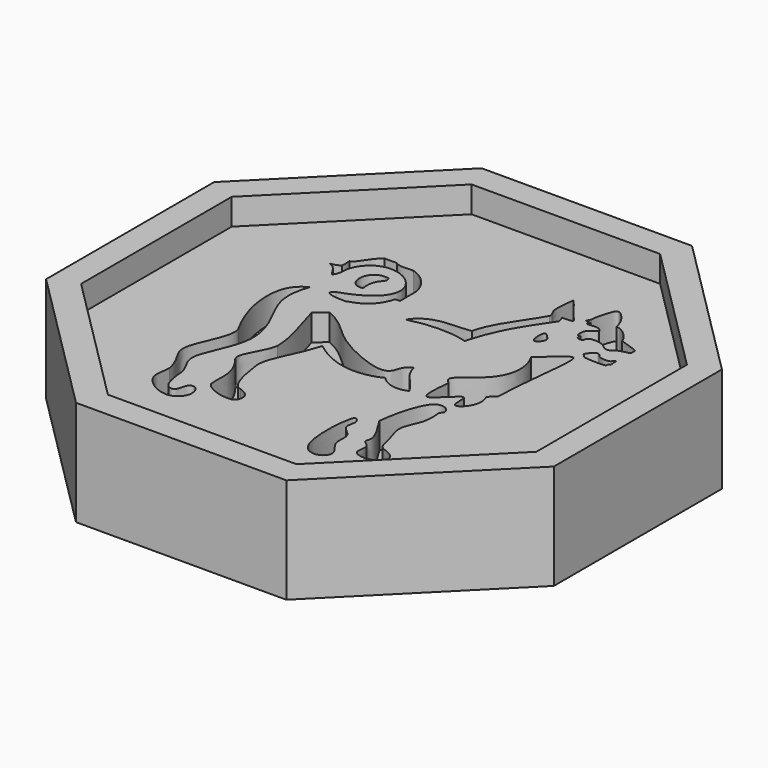
from build123d import *

# Parameters (mm, degrees)
F1_DEPTH = 25.4
F3_DEPTH = 6.35
F5_DEPTH = 6.35


with BuildPart() as f1:
    # F0 (on Top) → F1 (new body)
    with BuildSketch(Plane.XY):
        Polygon((-61.3372846899, 25.3607087968), (-61.3047391097, -25.4392807779), (-25.3607087968, -61.3372846899), (25.4392807779, -61.3047391097), (61.3372846899, -25.3607087968), (61.3047391097, 25.4392807779), (25.3607087968, 61.3372846899), (-25.4392807779, 61.3047391097), align=None)
    extrude(amount=F1_DEPTH)

    # F2 (on face) → F3 (cut)
    with BuildSketch(Plane.XY.offset(25.4)):
        Polygon((-54.9856008905, 22.734521413), (-54.9564255154, -22.8049569991), (-22.734521413, -54.9856008905), (22.8049569991, -54.9564255154), (54.9856008905, -22.734521413), (54.9564255154, 22.8049569991), (22.734521413, 54.9856008905), (-22.8049569991, 54.9564255154), align=None)
    extrude(amount=-F3_DEPTH, mode=Mode.SUBTRACT)

    # F4 (on face) → F5 (cut)
    with BuildSketch(Plane.XY.offset(19.05)):
        with BuildLine():
            add(Edge.make_bspline(
                [(-28.0372798443, 19.2676149309), (-28.8987054179, 20.3235540539), (-29.2879249901, 21.9352524728), (-31.1219263822, 22.5187968463)],
                knots=[0, 0, 0, 0, 4.4816546175, 4.4816546175, 4.4816546175, 4.4816546175], degree=3))
            add(Edge.make_bspline(
                [(-28.0372798443, 19.2676149309), (-26.9745588303, 20.3046072274), (-27.197111398, 22.6414259523), (-27.0301960409, 23.2191737741)],
                knots=[0, 0, 0, 0, 4.0778713907, 4.0778713907, 4.0778713907, 4.0778713907], degree=3))
            add(Edge.make_bspline(
                [(-27.0301960409, 23.2191737741), (-22.4121976644, 35.549569875), (-2.2154052276, 20.9722686559), (-22.9129437357, 14.1843669116)],
                knots=[0, 0, 0, 0, 9.9287210449, 9.9287210449, 9.9287210449, 9.9287210449], degree=3))
            add(Edge.make_bspline(
                [(-22.9129437357, 14.1843669116), (-25.3610387444, 12.6264877617), (-21.5219799429, 12.2926570475), (-19.185161218, 12.3482951894)],
                knots=[0, 0, 0, 0, 4.1554207811, 4.1554207811, 4.1554207811, 4.1554207811], degree=3))
            add(Edge.make_bspline(
                [(-19.185161218, 12.3482951894), (-16.6814271361, 13.1272347644), (-13.6213079095, 14.3512832001), (-12.3416194692, 18.8580043614)],
                knots=[0, 0, 0, 0, 9.4451245186, 9.4451245186, 9.4451245186, 9.4451245186], degree=3))
            add(Edge.make_bspline(
                [(-12.3416194692, 18.8580043614), (-11.9706960395, 18.8580043614), (-11.5997726098, 18.8580043614), (-11.22884918, 18.8580043614)],
                knots=[0, 0, 0, 0, 1.1127702892, 1.1127702892, 1.1127702892, 1.1127702892], degree=3))
            add(Edge.make_bspline(
                [(-11.22884918, 18.8580043614), (-11.22884918, 20.5086146792), (-11.22884918, 22.159224997), (-11.22884918, 23.8098353148)],
                knots=[0, 0, 0, 0, 4.9518309534, 4.9518309534, 4.9518309534, 4.9518309534], degree=3))
            add(Edge.make_bspline(
                [(-11.22884918, 23.8098353148), (-11.6183189675, 25.8128233254), (-13.0092836916, 28.7616662681), (-17.0152578503, 30.1526300609)],
                knots=[0, 0, 0, 0, 8.5856607487, 8.5856607487, 8.5856607487, 8.5856607487], degree=3))
            add(Edge.make_bspline(
                [(-17.0152578503, 30.1526300609), (-18.4618607163, 30.1526300609), (-20.2422942966, 29.7075212002), (-21.2994255126, 30.597737059)],
                knots=[0, 0, 0, 0, 4.3072279715, 4.3072279715, 4.3072279715, 4.3072279715], degree=3))
            add(Edge.make_bspline(
                [(-21.2994255126, 30.597737059), (-22.3009195179, 30.597737059), (-23.3024135232, 30.597737059), (-24.3039075285, 30.597737059)],
                knots=[0, 0, 0, 0, 3.004482016, 3.004482016, 3.004482016, 3.004482016], degree=3))
            add(Edge.make_bspline(
                [(-24.3039075285, 30.597737059), (-26.6407262534, 28.9842206985), (-27.4196658283, 25.8684623986), (-28.8662686944, 25.590268895)],
                knots=[0, 0, 0, 0, 6.77420673, 6.77420673, 6.77420673, 6.77420673], degree=3))
            add(Edge.make_bspline(
                [(-28.8662686944, 25.590268895), (-28.8662686944, 24.8484214147), (-28.5880770534, 24.0323897451), (-28.8662686944, 23.364726454)],
                knots=[0, 0, 0, 0, 2.225542441, 2.225542441, 2.225542441, 2.225542441], degree=3))
            add(Edge.make_bspline(
                [(-28.8662686944, 23.364726454), (-29.4782929122, 22.8083413094), (-30.3700404863, 22.6524043828), (-31.1219263822, 22.5187968463)],
                knots=[0, 0, 0, 0, 2.4090638235, 2.4090638235, 2.4090638235, 2.4090638235], degree=3))
        make_face()
        with BuildLine():
            add(Edge.make_bspline(
                [(-28.0008820709, 12.7586783027), (-29.8796463948, 7.5660265069), (-28.0287999384, 2.6821632246), (-26.7683431041, -0.0068068178), (-20.7281608533, -11.1412521717), (-29.5474328001, -23.7696430619), (-26.0852734071, -26.7943696783), (-25.2977338724, -29.1416380778)],
                knots=[0, 0, 0, 0, 0.2225477667, 0.3405641947, 0.5755616363, 0.8292797736, 1, 1, 1, 1], degree=3))
            add(Edge.make_bspline(
                [(-28.0008820709, 12.7586783027), (-29.4725771484, 11.8279191796), (-32.867634998, 9.2120678884), (-32.5076486915, -0.8590882644), (-28.0565619469, -8.8710384443)],
                knots=[0, 0, 0, 0, 0.3407457975, 1, 1, 1, 1], degree=3))
            add(Edge.make_bspline(
                [(-28.0565619469, -8.8710384443), (-26.4949586198, -11.4365298913), (-32.0736885782, -20.3703801564), (-30.4349170995, -24.4972697778), (-28.4926244503, -27.3833730072), (-28.0565638095, -29.6726982143)],
                knots=[0, 0, 0, 0, 0.4345714436, 0.6971037116, 1, 1, 1, 1], degree=3))
            add(Edge.make_bspline(
                [(-28.0565638095, -29.6726982143), (-28.0565638095, -31.237732619), (-29.6389633306, -35.0945037642), (-21.898898007, -39.9078726353), (-18.7092870474, -37.3579747975), (-18.3754581958, -35.6888175011)],
                knots=[0, 0, 0, 0, 0.316261051, 0.6980595292, 1, 1, 1, 1], degree=3))
            add(Edge.make_bspline(
                [(-18.3754581958, -35.6888175011), (-18.2647514631, -34.6924680256), (-18.4831757484, -33.6313286516), (-19.7782164584, -32.3324423498), (-21.4117624362, -33.3148451966), (-21.3484425752, -36.0815248294), (-24.3933898287, -36.1620581292), (-25.0957816794, -32.0893552414), (-25.2977338724, -29.1416380778)],
                knots=[0, 0, 0, 0, 0.1574034873, 0.285836077, 0.4154273106, 0.580633255, 0.7196315018, 1, 1, 1, 1], degree=3))
        make_face()
        with BuildLine():
            add(Edge.make_bspline(
                [(-18.7092870474, 6.9303079508), (-13.8535913481, 4.7580242148), (-11.9416435709, 0.119009405), (7.1841906574, -8.3140862474), (5.5491165258, -1.5267506242), (7.8859366477, -0.8590877987)],
                knots=[0, 0, 0, 0, 0.3593902316, 0.765142193, 1, 1, 1, 1], degree=3))
            add(Edge.make_bspline(
                [(-21.2686602026, 4.7580242148), (-20.4155358175, 5.4821187935), (-19.5624114325, 6.2062133721), (-18.7092870474, 6.9303079508)],
                knots=[0, 0, 0, 0, 3.3569640418, 3.3569640418, 3.3569640418, 3.3569640418], degree=3))
            add(Edge.make_bspline(
                [(-17.8190711886, -9.8725324497), (-17.9303474724, -6.0891113244), (-18.5980126262, -4.3086772785), (-21.2686602026, 4.7580242148)],
                knots=[0, 0, 0, 0, 15.0317281999, 15.0317281999, 15.0317281999, 15.0317281999], degree=3))
            add(Edge.make_bspline(
                [(-20.8235513419, -18.8859757036), (-21.713770926, -16.5491569787), (-18.3754581958, -13.6559531093), (-17.8190711886, -9.8725324497)],
                knots=[0, 0, 0, 0, 9.5010031199, 9.5010031199, 9.5010031199, 9.5010031199], degree=3))
            add(Edge.make_bspline(
                [(-17.9303487142, -29.8653164258), (-18.3754581958, -26.1189863086), (-16.8175771832, -24.0047220141), (-20.8235513419, -18.8859757036)],
                knots=[0, 0, 0, 0, 11.3541421577, 11.3541421577, 11.3541421577, 11.3541421577], degree=3))
            add(Edge.make_bspline(
                [(-17.262686044, -30.6813474745), (-17.4852402674, -30.4093371249), (-17.7077944908, -30.1373267753), (-17.9303487142, -29.8653164258)],
                knots=[0, 0, 0, 0, 1.0543624204, 1.0543624204, 1.0543624204, 1.0543624204], degree=3))
            add(Edge.make_bspline(
                [(-12.2552160174, -28.0106980354), (-11.2932488833, -28.3518757818), (-9.3914477485, -29.2781346218), (-9.8999895977, -32.4848488774), (-12.3449518616, -32.5252296346), (-14.7961370982, -32.1376830066), (-16.3743810316, -31.3027464304), (-17.262686044, -30.6813474745)],
                knots=[0, 0, 0, 0, 0.2134300381, 0.406934161, 0.5873424903, 0.7860112945, 1, 1, 1, 1], degree=3))
            add(Edge.make_bspline(
                [(-15.9273585305, -18.6634231359), (-15.3709752485, -22.780675441), (-14.4807593897, -27.788143605), (-12.2552160174, -28.0106980354)],
                knots=[0, 0, 0, 0, 10.0427176941, 10.0427176941, 10.0427176941, 10.0427176941], degree=3))
            add(Edge.make_bspline(
                [(-11.1424466595, -4.6425093897), (-13.0341565236, -11.096579954), (-16.2611911073, -14.7687252611), (-15.9273585305, -18.6634231359)],
                knots=[0, 0, 0, 0, 14.8149047885, 14.8149047885, 14.8149047885, 14.8149047885], degree=3))
            add(Edge.make_bspline(
                [(6.2167802826, -7.4244360439), (2.5446349755, -9.3161463737), (-4.1319923475, -10.3176408447), (-11.1424466595, -4.6425093897)],
                knots=[0, 0, 0, 0, 17.5807245566, 17.5807245566, 17.5807245566, 17.5807245566], degree=3))
            add(Edge.make_bspline(
                [(6.2167802826, -7.4244360439), (8.4423208609, -9.6499780193), (11.1129721627, -9.7612552345), (13.115959242, -8.7597612292)],
                knots=[0, 0, 0, 0, 7.0272159256, 7.0272159256, 7.0272159256, 7.0272159256], degree=3))
            add(Edge.make_bspline(
                [(7.8859366477, -0.8590877987), (8.7761525065, -4.5312321745), (11.3355256617, -5.5327252485), (13.115959242, -8.7597612292)],
                knots=[0, 0, 0, 0, 9.4749024792, 9.4749024792, 9.4749024792, 9.4749024792], degree=3))
        make_face()
        with BuildLine():
            add(Edge.make_bspline(
                [(-19.9287291616, 18.5597520322), (-20.7218211144, 23.2191737741), (-17.6485870034, 22.9217652231), (-18.6399519444, 24.7062239796)],
                knots=[0, 0, 0, 0, 6.2801324919, 6.2801324919, 6.2801324919, 6.2801324919], degree=3))
            add(Edge.make_bspline(
                [(-18.6399519444, 24.7062239796), (-23.9933300763, 25.8958619088), (-24.3898760527, 17.7666600794), (-19.9287291616, 18.5597520322)],
                knots=[0, 0, 0, 0, 6.2801324919, 6.2801324919, 6.2801324919, 6.2801324919], degree=3))
        make_face()
        with BuildLine():
            add(Edge.make_bspline(
                [(-5.6096651642, 13.6149282611), (-2.6132406574, 18.4601675352), (4.203310702, 17.065346241), (7.0364302956, 17.7666600802)],
                knots=[0, 0, 0, 0, 13.3101693256, 13.3101693256, 13.3101693256, 13.3101693256], degree=3))
            add(Edge.make_bspline(
                [(-5.6096651642, 13.6149282611), (1.4386394164, 15.3351114917), (6.2239428516, 14.3849765882), (8.5040840786, 13.6910192668)],
                knots=[0, 0, 0, 0, 14.1139543548, 14.1139543548, 14.1139543548, 14.1139543548], degree=3))
            add(Edge.make_bspline(
                [(8.5040840786, 13.6910192668), (10.7672957238, 22.0507318154), (14.4973509014, 26.6936998814), (17.3945371062, 31.0881678015)],
                knots=[0, 0, 0, 0, 19.537167967, 19.537167967, 19.537167967, 19.537167967], degree=3))
            add(Edge.make_bspline(
                [(16.957372427, 32.6494723558), (17.1044332286, 31.9786133866), (17.2474763046, 31.7590267708), (17.3945371062, 31.0881678015)],
                knots=[0, 0, 0, 0, 1.6213527895, 1.6213527895, 1.6213527895, 1.6213527895], degree=3))
            add(Edge.make_bspline(
                [(16.957372427, 32.6494723558), (17.6561995983, 32.5662349947), (18.8445488517, 32.710853988), (19.5890592956, 32.8586511932), (19.3132246383, 33.2443414188), (19.1744230688, 33.430121839)],
                knots=[0, 0, 0, 0, 0.4924790738, 0.7397762109, 1, 1, 1, 1], degree=3))
            add(Edge.make_bspline(
                [(14.147025533, 39.4879803061), (16.0163631663, 37.5952757895), (17.3050854355, 35.3228263557), (19.1744230688, 33.430121839)],
                knots=[0, 0, 0, 0, 7.8722535014, 7.8722535014, 7.8722535014, 7.8722535014], degree=3))
            add(Edge.make_bspline(
                [(14.6084949374, 31.7074209452), (14.8813206561, 32.4576937104), (13.1977047154, 33.5858091233), (14.0470692435, 37.3768965245), (14.147025533, 39.4879803061)],
                knots=[0, 0, 0, 0, 0.3731092448, 1, 1, 1, 1], degree=3))
            add(Edge.make_bspline(
                [(7.0364302956, 17.7666600802), (8.159278892, 22.8046998382), (12.0844733902, 27.0605006569), (14.6084949374, 31.7074209452)],
                knots=[0, 0, 0, 0, 15.8644563863, 15.8644563863, 15.8644563863, 15.8644563863], degree=3))
        make_face()
        with BuildLine():
            add(Edge.make_bspline(
                [(22.4148165435, 16.3930356503), (24.2836665154, 18.0725250896), (27.0029173159, 20.549754426), (30.4862581168, 22.5940611271), (27.8906989843, 10.1220104843), (27.6257377118, 0)],
                knots=[0, 0, 0, 0, 0.30682698, 0.451722506, 1, 1, 1, 1], degree=3))
            add(Edge.make_bspline(
                [(16.8506149203, -1.5367978485), (16.2638233056, -1.0676976254), (14.492191998, 0.4182380512), (24.3064990699, 5.4345626379), (24.4445025559, 13.0395053067), (22.4148165435, 16.3930356503)],
                knots=[0, 0, 0, 0, 0.1793899189, 0.5722506166, 1, 1, 1, 1], degree=3))
            add(Edge.make_bspline(
                [(25.9476453066, -1.5367978485), (27.8751199964, -5.0414433062), (21.9399501079, -11.1675266732), (24.2107532041, -0.8994806889), (15.6309805834, -12.4569427437), (16.5765762449, -5.1974706536), (16.8506149203, -1.5367978485)],
                knots=[0, 0, 0, 0, 0.2678703185, 0.4625212705, 0.7285866825, 1, 1, 1, 1], degree=3))
            add(Edge.make_bspline(
                [(27.6257377118, 0), (27.00749288, -0.3945002488), (26.5658901383, -1.1422975998), (25.9476453066, -1.5367978485)],
                knots=[0, 0, 0, 0, 2.2754651717, 2.2754651717, 2.2754651717, 2.2754651717], degree=3))
        make_face()
        with BuildLine():
            add(Edge.make_bspline(
                [(13.1382956089, -25.0052385354), (13.0518203589, -24.3990163752), (12.2797618583, -23.5602785403), (11.1105141174, -24.4906442838), (9.9794661919, -39.7643581614), (16.6902932342, -40.4762091746), (18.5003941614, -37.0816704912), (14.7121952101, -34.3856699364), (16.2425085179, -29.7885953701), (12.1334767397, -28.1036926101), (13.2568177087, -25.8361204735), (13.1382956089, -25.0052385354)],
                knots=[0, 0, 0, 0, 0.070863397, 0.1257912558, 0.3447714787, 0.4684229399, 0.5640410455, 0.6792790888, 0.7964704868, 0.9028753475, 1, 1, 1, 1], degree=3))
        make_face()
        with BuildLine():
            add(Edge.make_bspline(
                [(26.8536079675, -34.3594290316), (27.2714490269, -33.9821628087), (27.5024453322, -32.7005899885), (26.7680687179, -31.4202354743), (24.9856919844, -30.5617172645), (22.9394136433, -29.949434594), (22.5963966728, -25.9982062628), (20.4523282947, -21.7454574747), (23.4664017858, -17.1000129061), (23.2859773282, -13.901970828), (23.1107082218, -12.2754126787)],
                knots=[0, 0, 0, 0, 0.0942279731, 0.180240306, 0.2818144223, 0.3812242085, 0.5202976451, 0.6764919854, 0.8400809199, 1, 1, 1, 1], degree=3))
            add(Edge.make_bspline(
                [(23.1107082218, -12.2754126787), (23.3719449373, -11.9396689496), (24.0558658151, -11.4198851525), (23.0861654077, -9.7602822217), (21.0607759305, -9.4491379693), (18.8366493878, -10.9262737523), (16.9012901228, -16.7359576065), (16.3355525583, -21.8277908862)],
                knots=[0, 0, 0, 0, 0.1249392304, 0.2703068375, 0.4298225275, 0.6004042029, 1, 1, 1, 1], degree=3))
            add(Edge.make_bspline(
                [(16.3355525583, -21.8277908862), (18.0271967303, -24.4394007431), (20.4916306357, -28.2293568699), (18.9250976098, -30.2112847158), (21.7552155045, -31.1859912139), (20.0426765079, -34.8995275973), (24.030481665, -35.7434315914), (25.8822945146, -34.8796046714), (26.8536079675, -34.3594290316)],
                knots=[0, 0, 0, 0, 0.2587026579, 0.374487639, 0.5072905376, 0.6680701992, 0.8299419099, 1, 1, 1, 1], degree=3))
        make_face()
        with BuildLine():
            add(Edge.make_bspline(
                [(21.7349622399, 35.553496331), (21.7658607424, 37.0675561316), (22.4632394673, 38.882363824), (23.3020296061, 42.0712711659), (26.0613739336, 39.4891875495), (26.9902935393, 37.4381192754), (27.2932033986, 36.1467935145)],
                knots=[0, 0, 0, 0, 0.2771869874, 0.4887026549, 0.720573218, 1, 1, 1, 1], degree=3))
            add(Edge.make_bspline(
                [(21.7349622399, 35.553496331), (21.5371971329, 35.1371491949), (21.3394320259, 34.7208020588), (21.141666919, 34.3044549227)],
                knots=[0, 0, 0, 0, 1.3827884066, 1.3827884066, 1.3827884066, 1.3827884066], degree=3))
            add(Edge.make_bspline(
                [(21.141666919, 34.3044549227), (21.8087558435, 34.4154579868), (22.9192138443, 34.6067304975), (21.4795603217, 33.1570914073), (24.8269251292, 34.0492258481), (25.9508974805, 32.7494392023), (24.8371408796, 31.8640914709), (23.4804420172, 31.3425574603), (23.4607847126, 28.6895238735), (24.1020279011, 28.8438373479), (24.3267267942, 28.902342543)],
                knots=[0, 0, 0, 0, 0.125152921, 0.2174598066, 0.3898819729, 0.5128535986, 0.6270349481, 0.7586944031, 0.9155908851, 1, 1, 1, 1], degree=3))
            add(Edge.make_bspline(
                [(24.3267267942, 28.902342543), (24.2229816227, 28.6038598569), (23.9851884235, 27.9200704982), (26.085342966, 27.5495746546), (25.5276056432, 29.4944849548), (29.8622867299, 29.2394208692), (30.7261687198, 27.7118041566), (31.9865904748, 27.583418414), (32.6328612864, 27.9655586928)],
                knots=[0, 0, 0, 0, 0.1188505333, 0.272433173, 0.4094186307, 0.6538802305, 0.8270824788, 1, 1, 1, 1], degree=3))
            add(Edge.make_bspline(
                [(32.6328612864, 27.9655586928), (32.8335249786, 28.1902742706), (33.2336174509, 28.6383224955), (34.3439671713, 28.8890937502), (34.3502983451, 28.902342543)],
                knots=[0, 0, 0, 0, 0.460704687, 0.9185741337, 0.9185741337, 0.9185741337, 0.9185741337], degree=3))
            add(Edge.make_bspline(
                [(31.7412391305, 32.2801321745), (33.1424929006, 31.835327141), (35.226838432, 31.1736858282), (36.2862166852, 30.6450081764), (36.11125388, 30.0522757027), (36.2196886925, 29.168927145), (35.2529751699, 29.2132529834), (34.664836829, 29.0106795423), (34.3502983451, 28.902342543)],
                knots=[0, 0, 0, 0, 0.3086459553, 0.4591065741, 0.5732211024, 0.7057241065, 0.8426202018, 1, 1, 1, 1], degree=3))
            add(Edge.make_bspline(
                [(27.2932033986, 36.1467935145), (28.2362308353, 36.3459400833), (30.9350863099, 34.488286823), (31.7412391305, 32.2801321745)],
                knots=[0, 0, 0, 0, 5.8937332643, 5.8937332643, 5.8937332643, 5.8937332643], degree=3))
        make_face()
        with BuildLine():
            add(Edge.make_bspline(
                [(18.3871556073, 25.5505144596), (17.9028376551, 25.1303978825), (18.0261074441, 20.4826062167), (20.5294563919, 23.2130312074), (20.1078316388, 24.3166342383), (19.5788518638, 24.7728729875), (18.6807934383, 25.8052275461), (18.3871556073, 25.5505144596)],
                knots=[0, 0, 0, 0, 0.2957854791, 0.5149931194, 0.6764054606, 0.8206677945, 1, 1, 1, 1], degree=3))
        make_face()
        with BuildLine():
            add(Edge.make_bspline(
                [(31.0402363539, 25.4103131592), (30.4672511029, 25.1760278936), (29.104859761, 23.493828033), (29.6139441731, 23.3794331545), (30.143924243, 22.7198705463), (30.6213171009, 22.4392079924), (35.871355149, 22.2272396027), (35.5078651361, 22.8782942355), (35.8760179215, 23.1861553988), (36.263765113, 23.3794123673), (35.8971755298, 24.3484735935), (36.1899295548, 25.3338516374), (35.3340564337, 24.95144164), (35.4894175331, 24.1460136377), (32.4140667098, 24.1255824023), (32.1122134129, 25.1951283572), (31.6429421539, 25.2688406175), (31.3310553548, 25.5292247835), (31.0402363539, 25.4103131592)],
                knots=[0, 0, 0, 0, 0.1043569654, 0.1390084926, 0.196115789, 0.2536622599, 0.3977283401, 0.4333337447, 0.4763597791, 0.51537144, 0.5811685702, 0.6380204206, 0.6864109087, 0.7361998038, 0.8421424202, 0.9055749356, 0.9470335609, 1, 1, 1, 1], degree=3))
        make_face()
    extrude(amount=-F5_DEPTH, mode=Mode.SUBTRACT)


solid = f1.part
